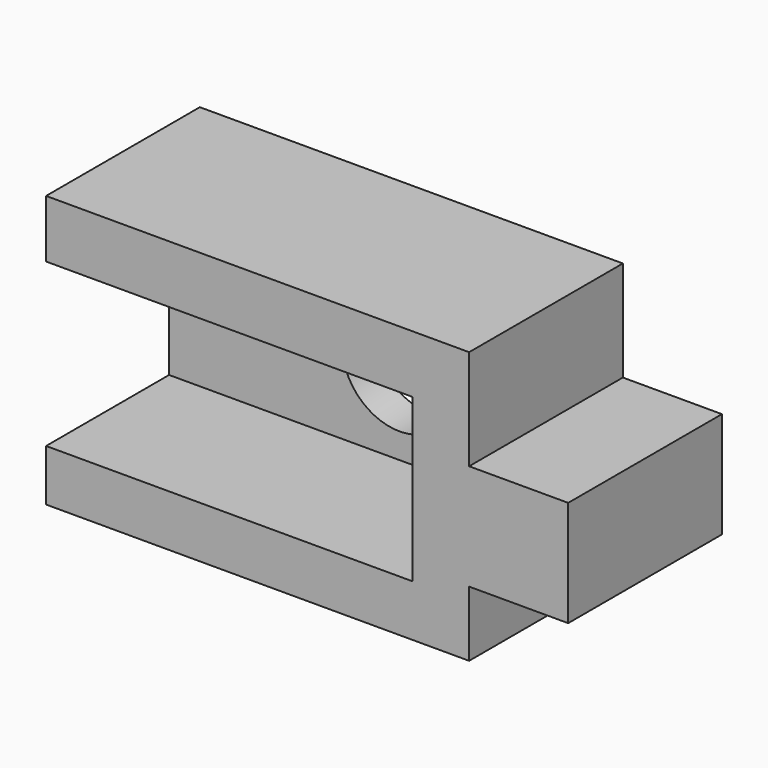
from build123d import *

# Parameters (mm, degrees)
F0_W     = 12.1704526246
F0_H     = 13.7812504545
F0_W_2   = 12.8863714635
F1_DEPTH = 25
F2_W     = 47.6974435151
F2_H     = 21.1193179712
F3_DEPTH = 20
F4_R     = 7.5
F5_DEPTH = 25


with BuildPart() as f1:
    # F0 (on Front) → F1 (new body)
    with BuildSketch(Plane.XZ):
        Polygon((0, 35.3480130434), (0, 0), (55.0355128944, 0), (55.0355128944, 8.5014207289), (42.8650602698, 8.5014207289), (42.8650602698, 22.2826711833), (55.0355128944, 22.2826711833), (55.0355128944, 35.3480130434), align=None)
        with Locations((48.9502865821, 15.3920459561)):
            Rectangle(F0_W, F0_H)
        with Locations((61.4786986262, 15.3920459561)):
            Rectangle(F0_W_2, F0_H)
    extrude(amount=F1_DEPTH)

    # F2 (on face) → F3 (cut)
    with BuildSketch(Plane.XZ.offset(25)):
        with Locations((23.8487217575, 17.2713068314)):
            Rectangle(F2_W, F2_H)
    extrude(amount=-F3_DEPTH, mode=Mode.SUBTRACT)

    # F4 (on face) → F5 (cut)
    with BuildSketch(Plane(origin=(0, 0, 0), x_dir=(-1, 0, 0), z_dir=(0, 1, 0))):
        with Locations((-30, 17.5)):
            Circle(F4_R)
    extrude(amount=-F5_DEPTH, mode=Mode.SUBTRACT)


solid = f1.part
